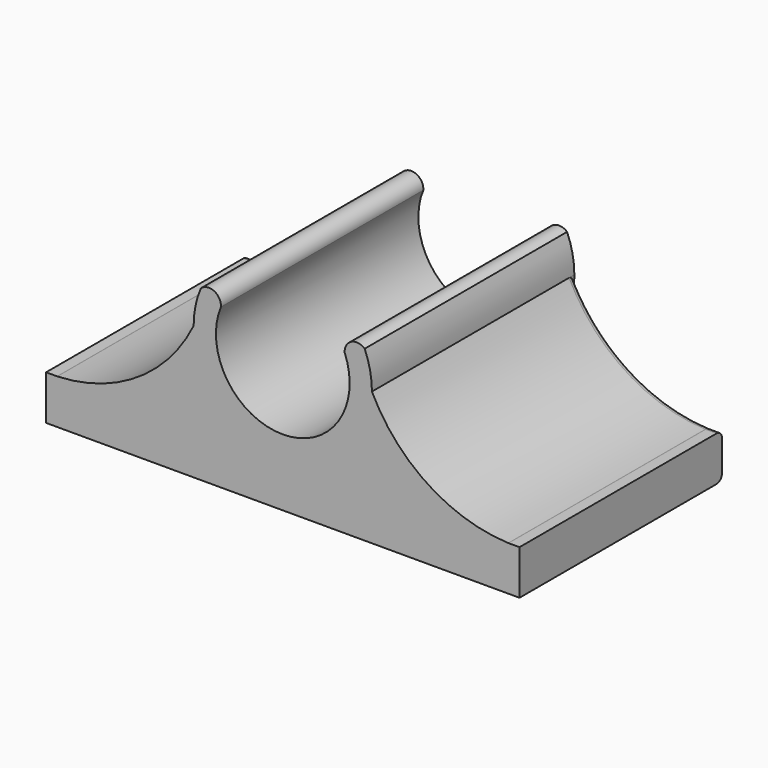
from build123d import *

# Parameters (mm, degrees)
F1_DEPTH     = 2
F3_DEPTH     = 40
F4_T1_DEPTH  = 40
F4_T3_DEPTH  = 90
F4_T5_DEPTH  = 20
F4_T8_ANGLE  = 90
F4_T10_ANGLE = 90
F4_T12_ANGLE = 90
F4_T14_ANGLE = 90
F4_T15_DEPTH = 20
F4_T17_DEPTH = 34.8706177507
F4_T19_DEPTH = 34.8706177507
F4_T22_ANGLE = 90
F4_T24_ANGLE = 90
F4_T26_ANGLE = 90
F4_T28_ANGLE = 90
F4_T32_ANGLE = 67.9058899257
F4_S33_R     = 4
F4_T34_DEPTH = 6
F4_T38_ANGLE = 67.9058899257
F4_S39_R     = 4
F4_T40_DEPTH = 6
F4_T42_ANGLE = 2.1985680139
F4_T44_ANGLE = 2.1985680139
F4_T46_ANGLE = 145.4380511244
F4_T48_ANGLE = 145.4380511244
F5_W         = 47.7962438017
F5_H         = 14.3843935803
F6_DEPTH     = 25
F7_W         = 52.0751457661
F7_H         = 31.3179213554
F8_DEPTH     = 25


# Not quite as in the source:
# - a fillet or chamfer that OpenCascade refuses, or shapes differently, is made with other operations: its cross-section is extruded or revolved along the edge and cut away or added


with BuildPart() as f1:
    # F0 (on Top) → F1 (new body)
    with BuildSketch(Plane.XY):
        with BuildLine():
            Line((45, 20), (-45, 20))
            ThreePointArc((-45, 20), (-52.0710678119, 17.0710678119), (-55, 10))
            Line((-55, 10), (-55, -10))
            ThreePointArc((-55, -10), (-52.0710678119, -17.0710678119), (-45, -20))
            Line((-45, -20), (45, -20))
            ThreePointArc((45, -20), (52.0710678119, -17.0710678119), (55, -10))
            Line((55, -10), (55, 10))
            ThreePointArc((55, 10), (52.0710678119, 17.0710678119), (45, 20))
        make_face()
    extrude(amount=F1_DEPTH)

    # F2 (on face) → F3 (join, through all)
    with BuildSketch(Plane(origin=(0, 20, 0), x_dir=(-1, 0, 0), z_dir=(0, 1, 0))):
        with BuildLine():
            ThreePointArc((2.7771054409, 7.1347622527), (0, 3), (-2.7771054409, 7.1347622527))
            ThreePointArc((-2.7771054409, 7.1347622527), (-3.0758368725, 7.6594328143), (-3.674432988, 7.5806777712))
            ThreePointArc((-3.674432988, 7.5806777712), (-3.9185059144, 6.8033127653), (-3.9999931862, 5.9926169097))
            ThreePointArc((-3.9999931862, 5.9926169097), (-6.509106512, 3.1485501635), (-10.1236877963, 2))
            Line((-10.1236877963, 2), (10.1236877963, 2))
            ThreePointArc((10.1236877963, 2), (6.509106512, 3.1485501635), (3.9999931862, 5.9926169097))
            ThreePointArc((3.9999931862, 5.9926169097), (3.9185059144, 6.8033127653), (3.674432988, 7.5806777712))
            ThreePointArc((3.674432988, 7.5806777712), (3.0758368725, 7.6594328143), (2.7771054409, 7.1347622527))
        make_face()
    extrude(amount=-F3_DEPTH)

    # F4: fillet of radius 0.3 on 22 edges, made by hand

    # F4_s2 → F4_t1 (join)
    with BuildSketch(Plane.XZ.offset(-20)):
        with BuildLine():
            ThreePointArc((10.1293822493, 2), (10.1236267648, 2.0000552144), (10.1178733989, 2.0002208373))
            ThreePointArc((10.1178733989, 2.0002208373), (10.120780575, 2.0001098236), (10.1236877963, 2))
            Line((10.1236877963, 2), (10.1293822493, 2))
        make_face()
        with BuildLine():
            ThreePointArc((-10.1293822493, 2), (-10.1236267648, 2.0000552144), (-10.1178733989, 2.0002208373))
            ThreePointArc((-10.1178733989, 2.0002208373), (-10.120780575, 2.0001098236), (-10.1236877963, 2))
            Line((-10.1236877963, 2), (-10.1293822493, 2))
        make_face()
    extrude(amount=F4_T1_DEPTH)

    # F4_s4 → F4_t3 (cut)
    with BuildSketch(Plane.YZ.offset(-45)):
        with BuildLine():
            ThreePointArc((20, 0.3), (19.9121320344, 0.0878679656), (19.7, 0))
            Line((19.7, 0), (20, 0))
            Line((20, 0), (20, 0.3))
        make_face()
        with BuildLine():
            ThreePointArc((-19.7, 0), (-19.9121320344, 0.0878679656), (-20, 0.3))
            Line((-20, 0.3), (-20, 0))
            Line((-20, 0), (-19.7, 0))
        make_face()
    extrude(amount=F4_T3_DEPTH, mode=Mode.SUBTRACT)

    # F4_s6 → F4_t5 (cut)
    with BuildSketch(Plane.XZ.offset(-10)):
        with BuildLine():
            ThreePointArc((-54.7, 0), (-54.9121320344, 0.0878679656), (-55, 0.3))
            Line((-55, 0.3), (-55, 0))
            Line((-55, 0), (-54.7, 0))
        make_face()
        with BuildLine():
            ThreePointArc((54.7, 0), (54.9121320344, 0.0878679656), (55, 0.3))
            Line((55, 0.3), (55, 0))
            Line((55, 0), (54.7, 0))
        make_face()
    extrude(amount=F4_T5_DEPTH, mode=Mode.SUBTRACT)

    # F4_s7 → F4_t8 (revolve, cut)
    with BuildSketch(Plane.YZ.offset(-45)):
        with BuildLine():
            ThreePointArc((20, 0.3), (19.9121320344, 0.0878679656), (19.7, 0))
            Line((19.7, 0), (20, 0))
            Line((20, 0), (20, 0.3))
        make_face()
    revolve(axis=Axis((-45, 10, 0), (0, 0, 1)), revolution_arc=F4_T8_ANGLE, mode=Mode.SUBTRACT)

    # F4_s9 → F4_t10 (revolve, cut)
    with BuildSketch(Plane.XZ.offset(10)):
        with BuildLine():
            ThreePointArc((-54.7, 0), (-54.9121320344, 0.0878679656), (-55, 0.3))
            Line((-55, 0.3), (-55, 0))
            Line((-55, 0), (-54.7, 0))
        make_face()
    revolve(axis=Axis((-45, -10, 0), (0, 0, 1)), revolution_arc=F4_T10_ANGLE, mode=Mode.SUBTRACT)

    # F4_s11 → F4_t12 (revolve, cut)
    with BuildSketch(Plane.YZ.offset(45)):
        with BuildLine():
            ThreePointArc((-19.7, 0), (-19.9121320344, 0.0878679656), (-20, 0.3))
            Line((-20, 0.3), (-20, 0))
            Line((-20, 0), (-19.7, 0))
        make_face()
    revolve(axis=Axis((45, -10, 0), (0, 0, 1)), revolution_arc=F4_T12_ANGLE, mode=Mode.SUBTRACT)

    # F4_s13 → F4_t14 (revolve, cut)
    with BuildSketch(Plane.XZ.offset(-10)):
        with BuildLine():
            ThreePointArc((55, 0.3), (54.9121320344, 0.0878679656), (54.7, 0))
            Line((54.7, 0), (55, 0))
            Line((55, 0), (55, 0.3))
        make_face()
    revolve(axis=Axis((45, 10, 0), (0, 0, 1)), revolution_arc=F4_T14_ANGLE, mode=Mode.SUBTRACT)

    # F4_s16 → F4_t15 (cut)
    with BuildSketch(Plane.XZ.offset(-10)):
        with BuildLine():
            ThreePointArc((54.7, 2), (54.9121320344, 1.9121320344), (55, 1.7))
            Line((55, 1.7), (55, 2))
            Line((55, 2), (54.7, 2))
        make_face()
        with BuildLine():
            ThreePointArc((-54.7, 2), (-54.9121320344, 1.9121320344), (-55, 1.7))
            Line((-55, 1.7), (-55, 2))
            Line((-55, 2), (-54.7, 2))
        make_face()
    extrude(amount=F4_T15_DEPTH, mode=Mode.SUBTRACT)

    # F4_s18 → F4_t17 (cut)
    with BuildSketch(Plane.YZ.offset(10.1293822493)):
        with BuildLine():
            ThreePointArc((-19.7, 2), (-19.9121320344, 1.9121320344), (-20, 1.7))
            Line((-20, 1.7), (-20, 2))
            Line((-20, 2), (-19.7, 2))
        make_face()
        with BuildLine():
            ThreePointArc((20, 1.7), (19.9121320344, 1.9121320344), (19.7, 2))
            Line((19.7, 2), (20, 2))
            Line((20, 2), (20, 1.7))
        make_face()
    extrude(amount=F4_T17_DEPTH, mode=Mode.SUBTRACT)

    # F4_s20 → F4_t19 (cut)
    with BuildSketch(Plane.YZ.offset(-45)):
        with BuildLine():
            ThreePointArc((-19.7, 2), (-19.9121320344, 1.9121320344), (-20, 1.7))
            Line((-20, 1.7), (-20, 2))
            Line((-20, 2), (-19.7, 2))
        make_face()
        with BuildLine():
            ThreePointArc((20, 1.7), (19.9121320344, 1.9121320344), (19.7, 2))
            Line((19.7, 2), (20, 2))
            Line((20, 2), (20, 1.7))
        make_face()
    extrude(amount=F4_T19_DEPTH, mode=Mode.SUBTRACT)

    # F4_s21 → F4_t22 (revolve, cut)
    with BuildSketch(Plane.XZ.offset(-10)):
        with BuildLine():
            ThreePointArc((54.7, 2), (54.9121320344, 1.9121320344), (55, 1.7))
            Line((55, 1.7), (55, 2))
            Line((55, 2), (54.7, 2))
        make_face()
    revolve(axis=Axis((45, 10, 2), (0, 0, 1)), revolution_arc=F4_T22_ANGLE, mode=Mode.SUBTRACT)

    # F4_s23 → F4_t24 (revolve, cut)
    with BuildSketch(Plane.YZ.offset(45)):
        with BuildLine():
            ThreePointArc((-19.7, 2), (-19.9121320344, 1.9121320344), (-20, 1.7))
            Line((-20, 1.7), (-20, 2))
            Line((-20, 2), (-19.7, 2))
        make_face()
    revolve(axis=Axis((45, -10, 2), (0, 0, 1)), revolution_arc=F4_T24_ANGLE, mode=Mode.SUBTRACT)

    # F4_s25 → F4_t26 (revolve, cut)
    with BuildSketch(Plane.XZ.offset(10)):
        with BuildLine():
            ThreePointArc((-54.7, 2), (-54.9121320344, 1.9121320344), (-55, 1.7))
            Line((-55, 1.7), (-55, 2))
            Line((-55, 2), (-54.7, 2))
        make_face()
    revolve(axis=Axis((-45, -10, 2), (0, 0, 1)), revolution_arc=F4_T26_ANGLE, mode=Mode.SUBTRACT)

    # F4_s27 → F4_t28 (revolve, cut)
    with BuildSketch(Plane.YZ.offset(-45)):
        with BuildLine():
            ThreePointArc((20, 1.7), (19.9121320344, 1.9121320344), (19.7, 2))
            Line((19.7, 2), (20, 2))
            Line((20, 2), (20, 1.7))
        make_face()
    revolve(axis=Axis((-45, 10, 2), (0, 0, 1)), revolution_arc=F4_T28_ANGLE, mode=Mode.SUBTRACT)


with BuildPart() as f4_tool30:
    # F4_s31 → F4_t32 (revolve)
    with BuildSketch(Plane(origin=(-1.7091793366, 0, 4.7227038559), x_dir=(0, 1, 0), z_dir=(-0.3403063894, 0, 0.9403146076))):
        with BuildLine():
            ThreePointArc((20, -5.4610241004), (19.9121320344, -5.6731561348), (19.7, -5.7610241004))
            Line((19.7, -5.7610241004), (20, -5.7610241004))
            Line((20, -5.7610241004), (20, -5.4610241004))
        make_face()
    revolve(axis=Axis((10.3905055755, 20, 9.1016638887), (0, -1, 0)), revolution_arc=F4_T32_ANGLE)

    # F4_s33 → F4_t34 (cut, symmetric)
    with BuildSketch(Plane.XZ.offset(-19.7)):
        with Locations((0, 6)):
            Circle(F4_S33_R)
    extrude(amount=F4_T34_DEPTH, both=True, mode=Mode.SUBTRACT)


with BuildPart() as f1_1:
    add(f1.part)

    # F4_t29: cut F4_tool30
    add(f4_tool30.part, mode=Mode.SUBTRACT)


with BuildPart() as f4_tool36:
    # F4_s37 → F4_t38 (revolve)
    with BuildSketch(Plane(origin=(-10.0263051977, 0, -0.3849208379), x_dir=(0, 1, 0), z_dir=(-0.9992638755, 0, -0.0383628346))):
        with BuildLine():
            ThreePointArc((20, -2.0868987298), (19.9121320344, -2.2990307641), (19.7, -2.3868987298))
            Line((19.7, -2.3868987298), (20, -2.3868987298))
            Line((20, -2.3868987298), (20, -2.0868987298))
        make_face()
    revolve(axis=Axis((-10.3905055755, 20, 9.1016638887), (0, -1, 0)), revolution_arc=F4_T38_ANGLE)

    # F4_s39 → F4_t40 (cut, symmetric)
    with BuildSketch(Plane.XZ.offset(-19.7)):
        with Locations((0, 6)):
            Circle(F4_S39_R)
    extrude(amount=F4_T40_DEPTH, both=True, mode=Mode.SUBTRACT)


with BuildPart() as f1_2:
    add(f1_1.part)

    # F4_t35: cut F4_tool36
    add(f4_tool36.part, mode=Mode.SUBTRACT)

    # F4_s41 → F4_t42 (revolve, cut)
    with BuildSketch(Plane.YZ.offset(-10.1293822493)):
        with BuildLine():
            ThreePointArc((20, 1.7), (19.9121320344, 1.9121320344), (19.7, 2))
            Line((19.7, 2), (20, 2))
            Line((20, 2), (20, 1.7))
        make_face()
    revolve(axis=Axis((-10.1293822493, 20, 2.3), (0, -1, 0)), revolution_arc=F4_T42_ANGLE, mode=Mode.SUBTRACT)

    # F4_s43 → F4_t44 (revolve, cut)
    with BuildSketch(Plane.YZ.offset(10.1293822493)):
        with BuildLine():
            ThreePointArc((20, 1.7), (19.9121320344, 1.9121320344), (19.7, 2))
            Line((19.7, 2), (20, 2))
            Line((20, 2), (20, 1.7))
        make_face()
    revolve(axis=Axis((10.1293822493, 20, 2.3), (0, 1, 0)), revolution_arc=F4_T44_ANGLE, mode=Mode.SUBTRACT)

    # F4_s45 → F4_t46 (revolve, cut)
    with BuildSketch(Plane.YZ.offset(-10.1293822493)):
        with BuildLine():
            ThreePointArc((-19.7, 2), (-19.9121320344, 1.9121320344), (-20, 1.7))
            Line((-20, 1.7), (-20, 2))
            Line((-20, 2), (-19.7, 2))
        make_face()
    revolve(axis=Axis((-10.1293822493, -20, 2.3), (0, -1, 0)), revolution_arc=F4_T46_ANGLE, mode=Mode.SUBTRACT)

    # F4_s47 → F4_t48 (revolve, cut)
    with BuildSketch(Plane.YZ.offset(10.1293822493)):
        with BuildLine():
            ThreePointArc((-19.7, 2), (-19.9121320344, 1.9121320344), (-20, 1.7))
            Line((-20, 1.7), (-20, 2))
            Line((-20, 2), (-19.7, 2))
        make_face()
    revolve(axis=Axis((10.1293822493, -20, 2.3), (0, 1, 0)), revolution_arc=F4_T48_ANGLE, mode=Mode.SUBTRACT)

    # F5 (on face) → F6 (cut)
    with BuildSketch(Plane.XY.offset(2)):
        with Locations((-34.5203755423, 13.9260510914)):
            Rectangle(F5_W, F5_H)
        Polygon((-10.6222536415, 6.7338543013), (-58.4184974432, 6.7338543013), (-58.4184974432, -28.1346440315), (65.8517405391, -28.1346440315), (65.8517405391, 6.7338543013), (58.4184974432, 6.7338543013), (10.6222536415, 6.7338543013), align=None)
        with Locations((34.5203755423, 13.9260510914)):
            Rectangle(F5_W, F5_H)
    extrude(amount=-F6_DEPTH, mode=Mode.SUBTRACT)

    # F7 (on Top) → F8 (cut)
    with BuildSketch(Plane.XY):
        with Locations((-5.8881500736, -7.0132566616)):
            Rectangle(F7_W, F7_H)
    extrude(amount=F8_DEPTH, mode=Mode.SUBTRACT)


solid = f1_2.part
